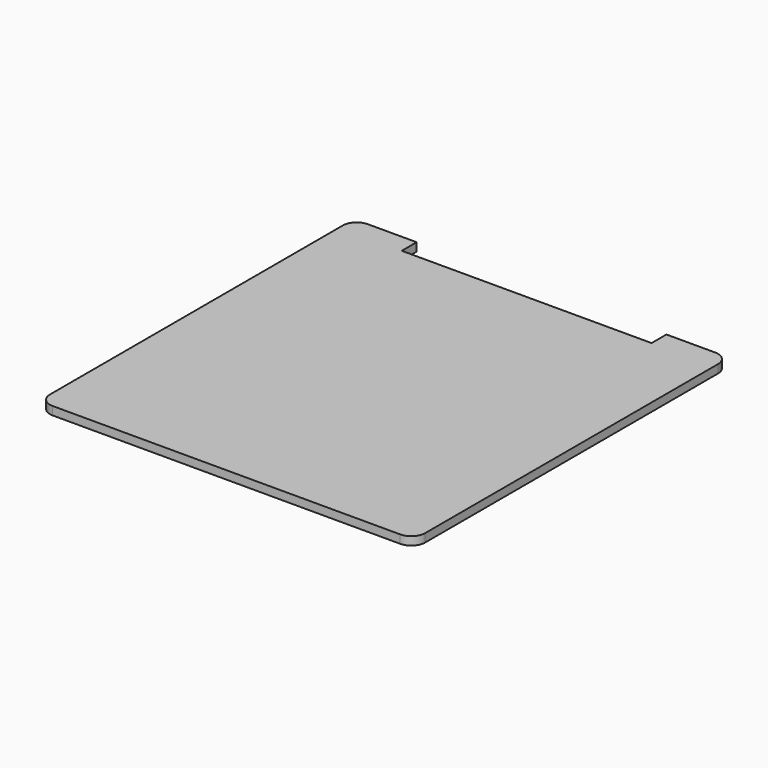
from build123d import *

# Parameters (mm, degrees)
F1_DEPTH = 18
F2_DEPTH = 12
F3_W     = 1252
F3_H     = 1252
F4_DEPTH = 18


with BuildPart() as f1:
    # F0 (on Top) → F1 (new body)
    with BuildSketch(Plane.XY):
        with BuildLine():
            Line((-626, -676), (626, -676))
            ThreePointArc((626, -676), (661.3553390593, -661.3553390593), (676, -626))
            Line((676, -626), (676, 626))
            Line((676, 626), (676, 693))
            ThreePointArc((676, 693), (661.3553390593, 728.3553390593), (626, 743))
            Line((626, 743), (450, 743))
            Line((450, 743), (450, 676))
            Line((450, 676), (-450, 676))
            Line((-450, 676), (-450, 743))
            Line((-450, 743), (-626, 743))
            ThreePointArc((-626, 743), (-661.3553390593, 728.3553390593), (-676, 693))
            Line((-676, 693), (-676, 626))
            Line((-676, 626), (-676, -626))
            ThreePointArc((-676, -626), (-661.3553390593, -661.3553390593), (-626, -676))
        make_face()
    extrude(amount=F1_DEPTH)

    # F2 (add): a face of the model
    f2_faces = [f1.faces().sort_by_distance(p)[0] for p in [
        (0, 11.5377812553, 18),
    ]]
    extrude(f2_faces, amount=F2_DEPTH)


with BuildPart() as f4:
    # F3 (on face) → F4 (new body)
    with BuildSketch(Plane(origin=(0, 0, 0), x_dir=(1, 0, 0), z_dir=(0, 0, -1))):
        Rectangle(F3_W, F3_H)
    extrude(amount=-F4_DEPTH)


with BuildPart() as f1_1:
    add(f1.part)

    # F5: cut F4
    add(f4.part, mode=Mode.SUBTRACT)


solid = Compound([f4.part, f1_1.part])
